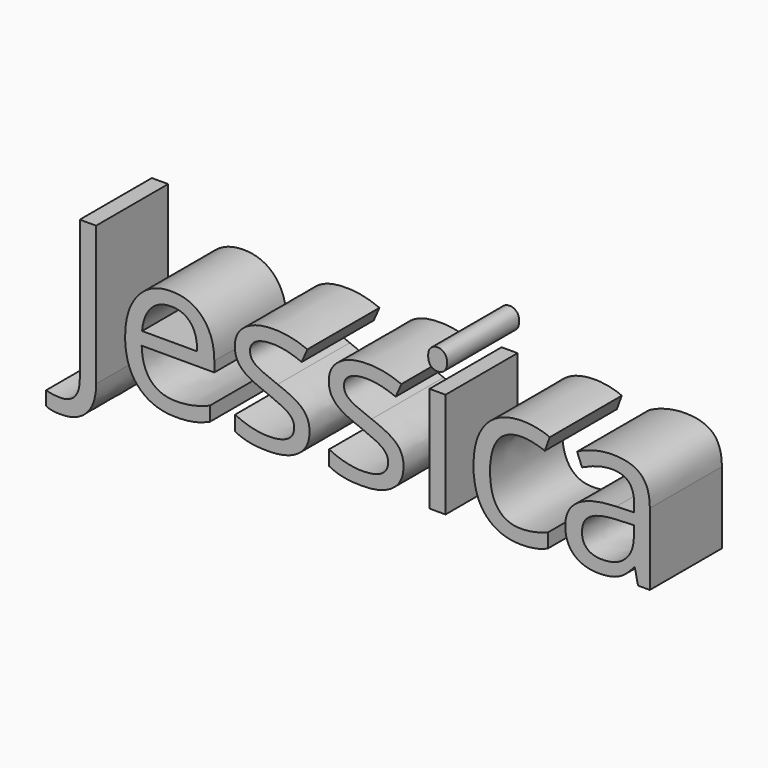
from build123d import *

# Parameters (mm, degrees)
F0_TEXT_SIZE = 13.8866249472
F1_DEPTH     = 6.35


# Not quite as in the source:
# - Text() gives the source's letters only with a copy of the font that has no kerning and outlines rounded to 1/6400 em; it was checked with that copy


with BuildPart() as f1:
    # F0 (on Front) → F1 (new body)
    with BuildSketch(Plane.XZ):
        with Locations((-13.365467079, 7.1602063254)):
            Text('Jessica', F0_TEXT_SIZE, font='Open Sans', text_align=(TextAlign.LEFT, TextAlign.BOTTOM))
    extrude(amount=F1_DEPTH)


solid = f1.part
